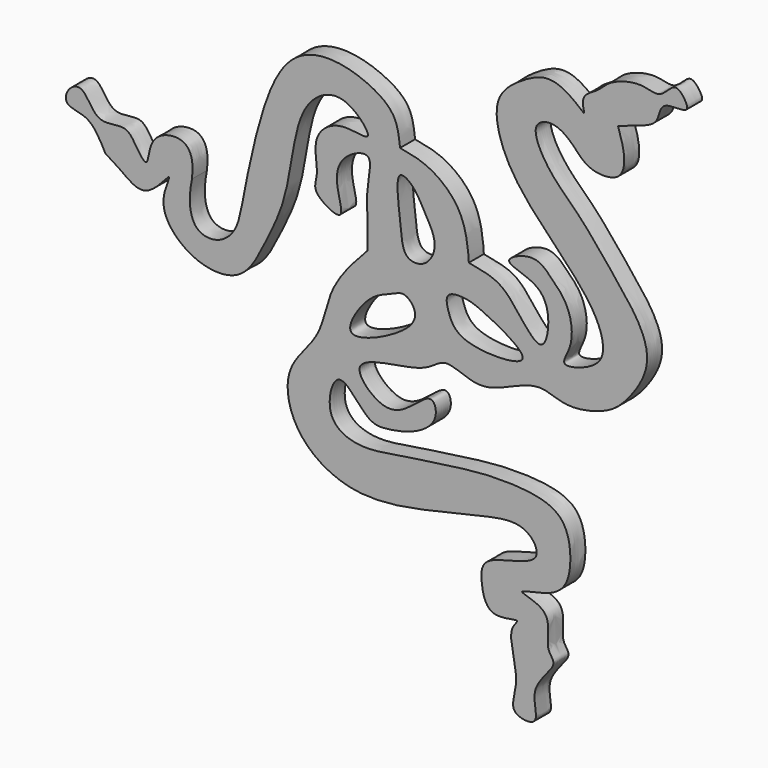
from build123d import *

# Parameters (mm, degrees)
F1_DEPTH = 2.5


with BuildPart() as f1:
    # F0 (on Front) → F1 (new body)
    with BuildSketch(Plane.XZ):
        with BuildLine():
            add(Edge.make_bspline(
                [(11.0889421776, 4.8053557985), (12.3664336611, 4.5789460208), (15.1323876511, 4.0887360773), (19.4792620619, 0.4607355169), (20.1712301772, -4.2707165664), (20.2260776558, -5.3110784429), (20.2452093363, -5.6739733554)],
                knots=[0, 0, 0, 0, 0.2633415775, 0.5701726363, 0.85006932, 1, 1, 1, 1], degree=3))
            add(Edge.make_bspline(
                [(11.0889421776, 4.8053557985), (10.9477114895, 6.0161080856), (10.6622771824, 8.4630992095), (7.5503208691, 10.8532625541), (2.4028051008, 12.5892131079), (-3.0144256065, 11.6772013784), (-7.1086081438, 5.5344278812), (-9.759717957, -7.3880363716), (-10.5372986967, -12.0565687383), (-13.1372199176, -14.3123320751), (-16.3285648842, -13.8978725755), (-17.1194246281, -10.625736306), (-16.7915869436, -8.7781875333), (-16.6287180036, -7.8603299335)],
                knots=[0, 0, 0, 0, 0.0795156219, 0.1607050617, 0.259282063, 0.3532252078, 0.4661828047, 0.6216277449, 0.7136151768, 0.7865258985, 0.8552481816, 0.9280876594, 1, 1, 1, 1], degree=3))
            add(Edge.make_bspline(
                [(-16.6287180036, -7.8603299335), (-16.5575606891, -7.1218084113), (-16.4149208991, -5.641390615), (-17.6041733535, -3.1201341795), (-22.513929949, -4.0988811412), (-22.3106075687, -8.9747043691), (-24.1376775807, -6.3798194605), (-25.389649227, -4.1422524297), (-29.4690409033, -5.8405928958), (-30.9664831344, -1.2725924402), (-33.3673187941, -2.583840604), (-33.6615781217, -4.8953370561), (-30.1398896289, -4.7830591729), (-28.8642099879, -7.243963074), (-28.1549822539, -8.612128906)],
                knots=[0, 0, 0, 0, 0.0759777977, 0.1523027839, 0.2532690375, 0.3427217753, 0.4113533356, 0.4905458161, 0.5831666784, 0.6791230306, 0.7482330679, 0.8126496123, 0.8958405491, 1, 1, 1, 1], degree=3))
            add(Edge.make_bspline(
                [(6.7823263817, -8.612128906), (6.8023463174, -7.6789212934), (6.8473800891, -5.5797208158), (6.4630197472, -1.4221142412), (7.7822890094, 3.471772956), (3.0761255876, 1.5106559717), (2.2591516242, -2.0872726175), (4.2492475431, -6.9934071521), (-0.9191321523, -4.1027508056), (0.4572576605, -1.9004592961), (-0.9264058685, 2.5984899734), (2.9858987401, 5.5912476588), (8.4322187338, 3.6876943929), (3.9069192717, 8.9116353995), (-0.4773551425, 7.4314984902), (-2.9869160352, 2.9560144756), (-3.7973868662, -5.9338096084), (-6.6805479463, -11.7120751903), (-9.6178927465, -17.8230555193), (-15.4445370698, -17.8676705477), (-19.6027912562, -14.9515606696), (-20.9677851586, -11.4707032937), (-18.7228290433, -6.9930832081), (-22.7039184604, -12.5660537681), (-25.8985798616, -9.9812289008), (-27.4312569811, -9.0512581458), (-28.1549822539, -8.612128906)],
                knots=[0, 0, 0, 0, 0.0355326697, 0.079928835, 0.1186755767, 0.1554413406, 0.1964473498, 0.2338421257, 0.2722447166, 0.3026401594, 0.3449488292, 0.3877259838, 0.4257202836, 0.4677010331, 0.5092484687, 0.554913877, 0.6163843036, 0.6704220242, 0.7215221279, 0.7678199717, 0.813448283, 0.8537725824, 0.8866164929, 0.9275861785, 0.9658064232, 1, 1, 1, 1], degree=3))
            add(Edge.make_bspline(
                [(40.1146747172, 16.7915038764), (40.4665507483, 15.7498959021), (41.1435519888, 13.745866561), (40.7189266585, 10.2344518158), (36.0130852525, 10.2326672231), (34.1986657339, 12.7738521997), (31.5413470961, 14.668522316), (28.1443108678, 13.4674789763), (30.9549521177, 8.1681167244), (34.8027089366, 5.0805254069), (40.124265207, -1.6001734888), (43.1761127371, -5.3964638729), (44.7381007749, -10.1648487415), (41.2943552054, -15.1875730535), (38.5918875439, -17.3957049024), (33.0828380013, -18.6445140842), (29.699042011, -16.5139924018), (24.9032970573, -18.9014914618), (21.1817394065, -20.0622987505), (16.7823866144, -17.5587003839), (14.6799623091, -20.8987623196), (2.7619930002, -21.1188631764), (8.8489886462, -27.1694642808), (12.3513095758, -25.4009682523), (15.4436882616, -22.3137079746), (16.3053064191, -25.7008071602), (13.2192577468, -28.0292088882), (9.4583495005, -28.7694708273), (6.5838065607, -28.8925602668), (2.694604328, -22.5961328405), (0.836620942, -29.9323358798), (5.315275849, -32.2886359905), (11.0487315026, -31.254668193), (20.2778131565, -29.8926966593), (24.5406386911, -29.6466323225), (29.9463342612, -29.9161495364), (33.4259529643, -31.8109051914), (34.1046432191, -37.0071173852), (32.5927705931, -41.2412291128), (25.0018643526, -41.8830302351), (31.7927394818, -42.766795317), (30.1346056521, -47.610502399), (32.5289051381, -49.0852212432), (27.8126248221, -52.5971654913), (30.243943881, -57.3093729522), (25.1455480434, -56.7072016872), (27.4240935302, -52.586613438), (25.0177552597, -46.9932134786), (27.6756341036, -45.0092103493), (22.7406737652, -46.7060028356), (21.8027202863, -42.5237815336), (21.9217264812, -38.9503862187), (30.7561795733, -38.4501545511), (27.9341960532, -33.5796496944), (22.1150849746, -34.697382944), (15.0103365649, -36.5180323369), (4.8269707459, -38.4537896904), (-3.1884442224, -33.6458748824), (-4.7785630469, -25.6299041474), (0.8111431792, -21.0494402895), (1.400351515, -14.3931754671), (4.9253784653, -10.6067689094), (6.7823263817, -8.612128906)],
                knots=[0, 0, 0, 0, 0.0143343431, 0.0275789403, 0.0427717568, 0.0567220329, 0.07059303, 0.0826300691, 0.099771732, 0.1183160944, 0.1411505414, 0.1588376485, 0.1755638368, 0.1942322152, 0.2092904681, 0.2272516601, 0.2424083772, 0.2599391332, 0.2756498287, 0.2914865856, 0.3064153176, 0.3295241271, 0.346342083, 0.3619353534, 0.3762163746, 0.3872662203, 0.4022304726, 0.4176973024, 0.4309009199, 0.4482919704, 0.4647186379, 0.4807613357, 0.5001067849, 0.5241273741, 0.5409051779, 0.5588572741, 0.5737869973, 0.5910192967, 0.6075380946, 0.6240349255, 0.6383527412, 0.65428164, 0.6647212347, 0.6816370716, 0.6966872857, 0.7093429575, 0.7243931718, 0.7436387934, 0.7529292754, 0.7668217904, 0.7815692023, 0.7951918317, 0.8155415987, 0.8291012376, 0.8474135009, 0.8693670546, 0.8944821747, 0.9175158167, 0.9381534048, 0.9582127435, 0.9779869034, 1, 1, 1, 1], degree=3))
            add(Edge.make_bspline(
                [(35.6215797365, 16.7915038764), (35.4699922434, 17.5248150308), (35.1615979616, 19.0166859113), (37.5471970561, 20.0044705983), (38.7922008862, 21.7367388394), (43.1261085049, 23.0809638555), (45.7430187509, 21.666539652), (47.5175099347, 24.3510448141), (48.8499940298, 23.209644854), (49.9676665537, 21.0588237026), (45.5578001356, 21.9270429172), (45.7094218616, 18.6229828126), (42.5187291989, 17.7018461176), (40.9018023392, 17.0895651429), (40.1146747172, 16.7915038764)],
                knots=[0, 0, 0, 0, 0.0761907285, 0.1550047733, 0.2349555648, 0.3459562777, 0.4329552921, 0.5157211357, 0.5792215223, 0.6442301631, 0.7366502925, 0.8196012258, 0.9121810258, 1, 1, 1, 1], degree=3))
            add(Edge.make_bspline(
                [(20.2452093363, -5.6739733554), (21.6511226884, -5.919978834), (24.4468348201, -6.4091700773), (26.7096769623, -9.2666795713), (30.1425392507, -13.6985972103), (31.1948008112, -8.8504492738), (30.0135648348, -5.2465348991), (26.2482784161, -4.3943314402), (25.0663521703, -3.4474039969), (29.0052041471, -1.6430971727), (31.273426782, -3.9254865804), (33.70859268, -6.3528940117), (34.3599178917, -10.8674365497), (31.8004493289, -14.225787817), (37.3041746939, -12.6218900027), (38.561871108, -9.9219512268), (36.8702090159, -5.134584014), (30.6844857187, 1.0727408413), (25.0457946051, 7.2338592725), (23.0617147536, 14.7304713584), (26.9116572333, 17.8795520359), (30.3337468395, 19.6926905477), (33.15171401, 18.8464314896), (34.7729102644, 17.4975966466), (35.6215797365, 16.7915038764)],
                knots=[0, 0, 0, 0, 0.0465105549, 0.0924880061, 0.1380869348, 0.1791743014, 0.2240340473, 0.2680243733, 0.2884436799, 0.3299757418, 0.3700060981, 0.4127382408, 0.4618481436, 0.4976734906, 0.5429073579, 0.5814208302, 0.6307280454, 0.6995088401, 0.7679009824, 0.827826658, 0.8762547925, 0.9207954542, 0.958537728, 1, 1, 1, 1], degree=3))
        make_face()
        with BuildLine():
            add(Edge.make_bspline(
                [(4.6297861263, -18.9531669021), (3.8919879115, -18.2827722332), (6.7824732199, -13.636765733), (9.6478068057, -12.9329740097), (11.5968616577, -11.7570107669), (13.379785524, -13.5277113185), (12.8210888596, -16.4351768322), (5.5558528159, -19.7946302714), (4.6297861263, -18.9531669021)],
                knots=[0, 0, 0, 0, 0.1990242948, 0.3624068162, 0.4835167179, 0.6045300721, 0.7501894608, 1, 1, 1, 1], degree=3))
        make_face(mode=Mode.SUBTRACT)
        with BuildLine():
            add(Edge.make_bspline(
                [(27.3912567645, -14.6327018738), (27.7337695891, -13.7304643049), (22.4200581125, -10.8118886708), (19.875056693, -9.848919268), (16.9580902342, -10.0392418511), (17.5734112898, -12.7084904983), (19.1166314264, -15.8012985206), (27.0018422056, -15.6584866614), (27.3912567645, -14.6327018738)],
                knots=[0, 0, 0, 0, 0.2040340369, 0.3652437321, 0.4873603759, 0.6082438326, 0.7680267166, 1, 1, 1, 1], degree=3))
        make_face(mode=Mode.SUBTRACT)
        with BuildLine():
            add(Edge.make_bspline(
                [(11.0889421776, 1.5953831607), (10.4635155898, 1.0790307729), (11.2049354821, -3.9801423175), (11.4095818962, -8.1387584169), (14.6867009262, -8.1070749026), (16.2991242757, -4.9079617981), (14.3654117825, -1.7822196639), (13.0389671009, 0.9354236274), (11.4379506775, 1.8835246882), (11.0889421776, 1.5953831607)],
                knots=[0, 0, 0, 0, 0.1852845465, 0.3457701949, 0.4646652511, 0.6024119976, 0.7519992867, 0.8966051605, 1, 1, 1, 1], degree=3))
        make_face(mode=Mode.SUBTRACT)
    extrude(amount=F1_DEPTH)


solid = f1.part
